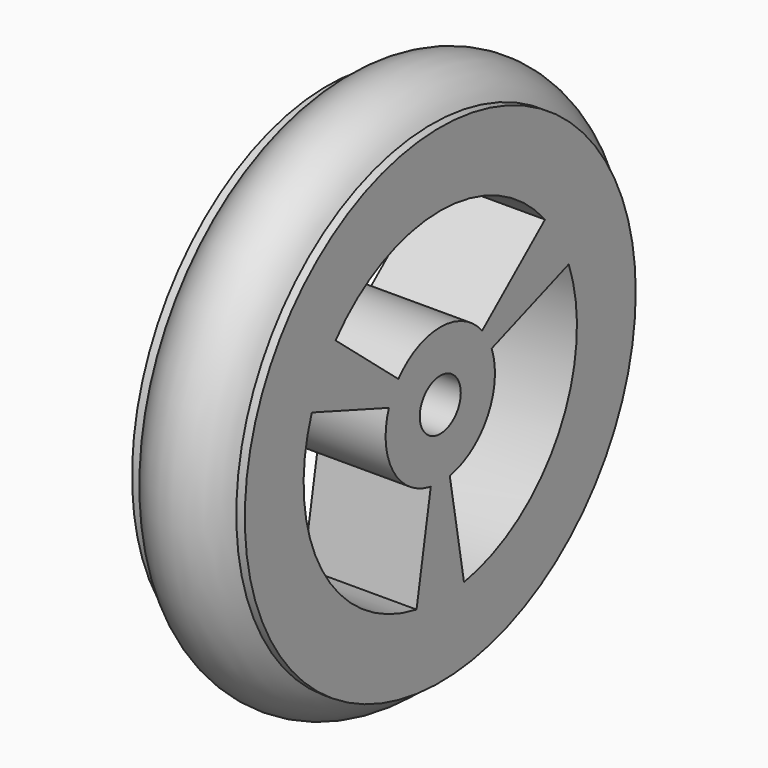
from build123d import *

# Parameters (mm, degrees)
F2_R            = 1.5
F3_DEPTH        = 25
F3_COPIES_COUNT = 3


# Not quite as in the source:
# - a pattern or mirror of a feature is missing from the dataset's text; its kind, count and spacing are read off the source's solid


with BuildPart() as f1:
    # F0 (on Top) → F1 (revolve)
    with BuildSketch(Plane.XY):
        with BuildLine():
            Line((0, 3), (0, 0))
            Line((0, 0), (8.6, 0))
            Line((8.6, 0), (8.6, 14.3))
            Line((8.6, 14.3), (8.1, 14.3))
            ThreePointArc((8.1, 14.3), (5.3, 16), (2.5, 14.3))
            Line((2.5, 14.3), (2, 14.3))
            Line((2, 14.3), (2, 3))
            Line((2, 3), (0, 3))
        make_face()
    revolve(axis=Axis((4.3, 0, 0), (-1, 0, 0)))

    # F2 (on face) → F3 (cut)
    with BuildSketch(Plane.YZ.offset(8.6)):
        Circle(F2_R)
        with BuildLine():
            ThreePointArc((-3.0641777725, 2.5711504387), (0, 4), (3.0641777725, 2.5711504387))
            Line((3.0641777725, 2.5711504387), (7.6604444312, 6.4278760969))
            ThreePointArc((7.6604444312, 6.4278760969), (0, 10), (-7.6604444312, 6.4278760969))
            Line((-7.6604444312, 6.4278760969), (-3.0641777725, 2.5711504387))
        make_face()
    f3 = extrude(amount=-F3_DEPTH, mode=Mode.SUBTRACT)

    # F3_copies: F3 ×3 about axis
    f3_copies_axis = Axis((0, 0, 0), (1, 0, 0))
    for i in range(1, F3_COPIES_COUNT):
        add(f3.rotate(f3_copies_axis, i * 360 / F3_COPIES_COUNT), mode=Mode.SUBTRACT)


solid = f1.part
